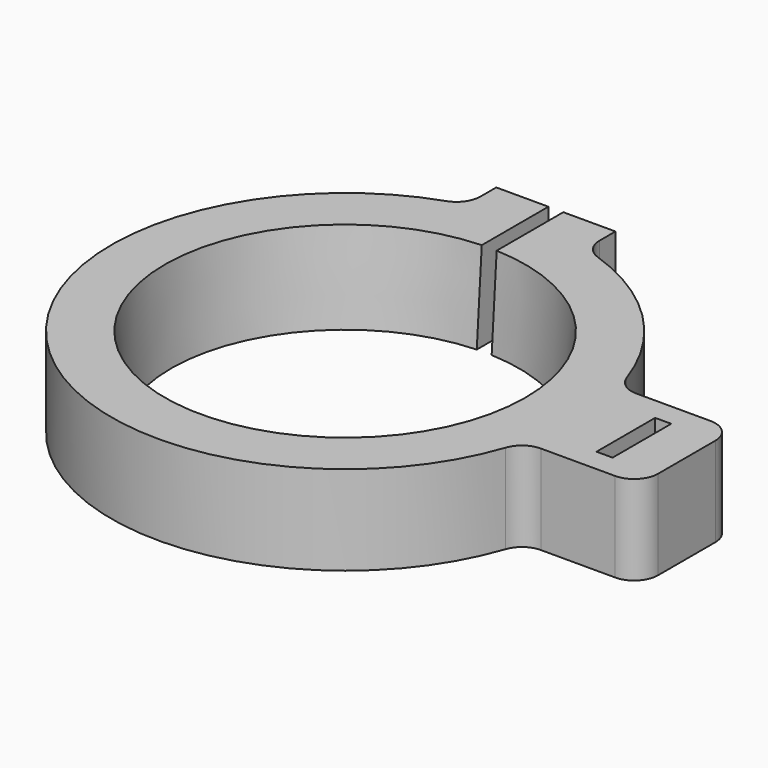
from build123d import *

# Parameters (mm, degrees)
F0_R           = 49.784
F0_R_2         = 37.084
F1_DEPTH       = 19.05
F2_R           = 37.084
F3_DEPTH       = 19.05
F3_TAPER       = -4
F4_W           = 25.4
F4_H           = 17.7178942325
F5_DEPTH       = 19.05
F6_W           = 3.175
F6_H           = 19.0839946053
F7_DEPTH       = 19.0510001
F8_W           = 34.3662
F8_H           = 25.4
F9_DEPTH       = 19.05
F10_W          = 3.429
F10_H          = 15.621
F11_DEPTH      = 19.0510001
F12_R          = 2.5527
F13_DEPTH      = 11.1125
F13_DEPTH_BACK = 60.0833057675
F14_R          = 5.5245
F15_DEPTH      = 3.175
F15_DEPTH_BACK = 60.0833057675
F17_D          = 3.7973
F18_T1_DEPTH   = 19.05
F18_T6_DEPTH   = 13.4160756928
F18_S7_R       = 5.5245
F18_T8_DEPTH   = 9
F18_T12_DEPTH  = 13.4160756928
F18_S13_R      = 5.5245
F18_T14_DEPTH  = 9
F18_T18_DEPTH  = 17.0419256928
F18_S19_R      = 1.89865
F18_T20_DEPTH  = 11
F18_T24_DEPTH  = 17.0419256928
F18_S25_R      = 1.89865
F18_T26_DEPTH  = 11
F18_T27_DEPTH  = 44.45


# Not quite as in the source:
# - a fillet or chamfer that OpenCascade refuses, or shapes differently, is made with other operations: its cross-section is extruded or revolved along the edge and cut away or added


with BuildPart() as f1:
    # F0 (on Top) → F1 (new body)
    with BuildSketch(Plane.XY):
        Circle(F0_R)
        Circle(F0_R_2, mode=Mode.SUBTRACT)
    extrude(amount=F1_DEPTH)

    # F2 (on face) → F3 (cut)
    with BuildSketch(Plane(origin=(0, 0, 0), x_dir=(1, 0, 0), z_dir=(0, 0, -1))):
        Circle(F2_R)
    extrude(amount=-F3_DEPTH, taper=F3_TAPER, mode=Mode.SUBTRACT)

    # F4 (on face) → F5 (join)
    with BuildSketch(Plane.XY.offset(19.05)):
        with Locations((0, 47.2750528838)):
            Rectangle(F4_W, F4_H)
    extrude(amount=-F5_DEPTH)

    # F6 (on face) → F7 (cut, through all)
    with BuildSketch(Plane.XY.offset(19.05)):
        with Locations((0, 46.5920026974)):
            Rectangle(F6_W, F6_H)
    extrude(amount=-F7_DEPTH, mode=Mode.SUBTRACT)

    # F8 (on face) → F9 (join)
    with BuildSketch(Plane.XY.offset(19.05)):
        with Locations((55.5992057675, 0)):
            Rectangle(F8_W, F8_H)
    extrude(amount=-F9_DEPTH)

    # F10 (on face) → F11 (cut, through all)
    with BuildSketch(Plane.XY.offset(19.05)):
        with Locations((61.5315, 0)):
            Rectangle(F10_W, F10_H)
    extrude(amount=-F11_DEPTH, mode=Mode.SUBTRACT)

    # F12 (on face) → F13 (cut, two sides)
    with BuildSketch(Plane.YZ.offset(12.7)) as f13_sk:
        with Locations((48.1368534078, 9.525)):
            Circle(F12_R)
    extrude(amount=-F13_DEPTH, mode=Mode.SUBTRACT)
    extrude(f13_sk.sketch, amount=F13_DEPTH_BACK, mode=Mode.SUBTRACT)

    # F14 (on face) → F15 (cut, two sides)
    with BuildSketch(Plane.YZ.offset(12.7)) as f15_sk:
        with Locations((48.1368534078, 9.525)):
            Circle(F14_R)
    extrude(amount=-F15_DEPTH, mode=Mode.SUBTRACT)
    extrude(f15_sk.sketch, amount=F15_DEPTH_BACK, mode=Mode.SUBTRACT)

    # F17 (through all)
    with Locations(Plane.YZ.offset(-1.5875)):
        with Locations((48.1368534078, 9.525)):
            Hole(F17_D / 2)

    # F18: fillet of radius 5.08 on 8 edges, made by hand

    # F18_s2 → F18_t1 (join)
    with BuildSketch(Plane.XY):
        with BuildLine():
            ThreePointArc((47.0972426029, -16.1337037037), (48.949846917, -13.6466245522), (51.9030836849, -12.7))
            Line((51.9030836849, -12.7), (48.1368534078, -12.7))
            ThreePointArc((48.1368534078, -12.7), (47.6479888455, -14.4262197049), (47.0972426029, -16.1337037037))
        make_face()
        with BuildLine():
            ThreePointArc((51.9030836849, 12.7), (48.949846917, 13.6466245522), (47.0972426029, 16.1337037037))
            ThreePointArc((47.0972426029, 16.1337037037), (47.6479888455, 14.4262197049), (48.1368534078, 12.7))
            Line((48.1368534078, 12.7), (51.9030836849, 12.7))
        make_face()
    extrude(amount=F18_T1_DEPTH)


with BuildPart() as f18_tool4:
    # F18_s5 → F18_t6 (new body)
    with BuildSketch(Plane.XY.offset(13.4160756928)):
        with BuildLine():
            ThreePointArc((12.7, 51.9030836849), (13.6466245522, 48.949846917), (16.1337037037, 47.0972426029))
            ThreePointArc((16.1337037037, 47.0972426029), (14.4262197049, 47.6479888455), (12.7, 48.1368534078))
            Line((12.7, 48.1368534078), (12.7, 51.9030836849))
        make_face()
    extrude(amount=-F18_T6_DEPTH)

    # F18_s7 → F18_t8 (cut, symmetric)
    with BuildSketch(Plane.YZ.offset(14.4)):
        with Locations((48.1368534078, 9.525)):
            Circle(F18_S7_R)
    extrude(amount=F18_T8_DEPTH, both=True, mode=Mode.SUBTRACT)


with BuildPart() as f1_1:
    add(f1.part)

    # F18_t3: union F18_tool4
    add(f18_tool4.part)


with BuildPart() as f18_tool10:
    # F18_s11 → F18_t12 (new body)
    with BuildSketch(Plane.XY.offset(19.05)):
        with BuildLine():
            ThreePointArc((12.7, 51.9030836849), (13.6466245522, 48.949846917), (16.1337037037, 47.0972426029))
            ThreePointArc((16.1337037037, 47.0972426029), (14.4262197049, 47.6479888455), (12.7, 48.1368534078))
            Line((12.7, 48.1368534078), (12.7, 51.9030836849))
        make_face()
    extrude(amount=-F18_T12_DEPTH)

    # F18_s13 → F18_t14 (cut, symmetric)
    with BuildSketch(Plane.YZ.offset(14.4)):
        with Locations((48.1368534078, 9.525)):
            Circle(F18_S13_R)
    extrude(amount=F18_T14_DEPTH, both=True, mode=Mode.SUBTRACT)


with BuildPart() as f1_2:
    add(f1_1.part)

    # F18_t9: union F18_tool10
    add(f18_tool10.part)


with BuildPart() as f18_tool16:
    # F18_s17 → F18_t18 (new body)
    with BuildSketch(Plane.XY.offset(19.05)):
        with BuildLine():
            ThreePointArc((-16.1337037037, 47.0972426029), (-13.6466245522, 48.949846917), (-12.7, 51.9030836849))
            Line((-12.7, 51.9030836849), (-12.7, 48.1368534078))
            ThreePointArc((-12.7, 48.1368534078), (-14.4262197049, 47.6479888455), (-16.1337037037, 47.0972426029))
        make_face()
    extrude(amount=-F18_T18_DEPTH)

    # F18_s19 → F18_t20 (cut, symmetric)
    with BuildSketch(Plane.YZ.offset(-14.4)):
        with Locations((48.1368534078, 9.525)):
            Circle(F18_S19_R)
    extrude(amount=F18_T20_DEPTH, both=True, mode=Mode.SUBTRACT)


with BuildPart() as f1_3:
    add(f1_2.part)

    # F18_t15: union F18_tool16
    add(f18_tool16.part)


with BuildPart() as f18_tool22:
    # F18_s23 → F18_t24 (new body)
    with BuildSketch(Plane.XY.offset(17.0419256928)):
        with BuildLine():
            ThreePointArc((-16.1337037037, 47.0972426029), (-13.6466245522, 48.949846917), (-12.7, 51.9030836849))
            Line((-12.7, 51.9030836849), (-12.7, 48.1368534078))
            ThreePointArc((-12.7, 48.1368534078), (-14.4262197049, 47.6479888455), (-16.1337037037, 47.0972426029))
        make_face()
    extrude(amount=-F18_T24_DEPTH)

    # F18_s25 → F18_t26 (cut, symmetric)
    with BuildSketch(Plane.YZ.offset(-14.4)):
        with Locations((48.1368534078, 9.525)):
            Circle(F18_S25_R)
    extrude(amount=F18_T26_DEPTH, both=True, mode=Mode.SUBTRACT)


with BuildPart() as f1_4:
    add(f1_3.part)

    # F18_t21: union F18_tool22
    add(f18_tool22.part)

    # F18_s28 → F18_t27 (cut)
    with BuildSketch(Plane.XY.offset(-12.7)):
        with BuildLine():
            ThreePointArc((67.7023057675, -12.7), (71.294408216, -11.2121024484), (72.7823057675, -7.62))
            Line((72.7823057675, -7.62), (72.7823057675, -12.7))
            Line((72.7823057675, -12.7), (67.7023057675, -12.7))
        make_face()
        with BuildLine():
            ThreePointArc((72.7823057675, 7.62), (71.294408216, 11.2121024484), (67.7023057675, 12.7))
            Line((67.7023057675, 12.7), (72.7823057675, 12.7))
            Line((72.7823057675, 12.7), (72.7823057675, 7.62))
        make_face()
    extrude(amount=F18_T27_DEPTH, mode=Mode.SUBTRACT)


solid = f1_4.part
